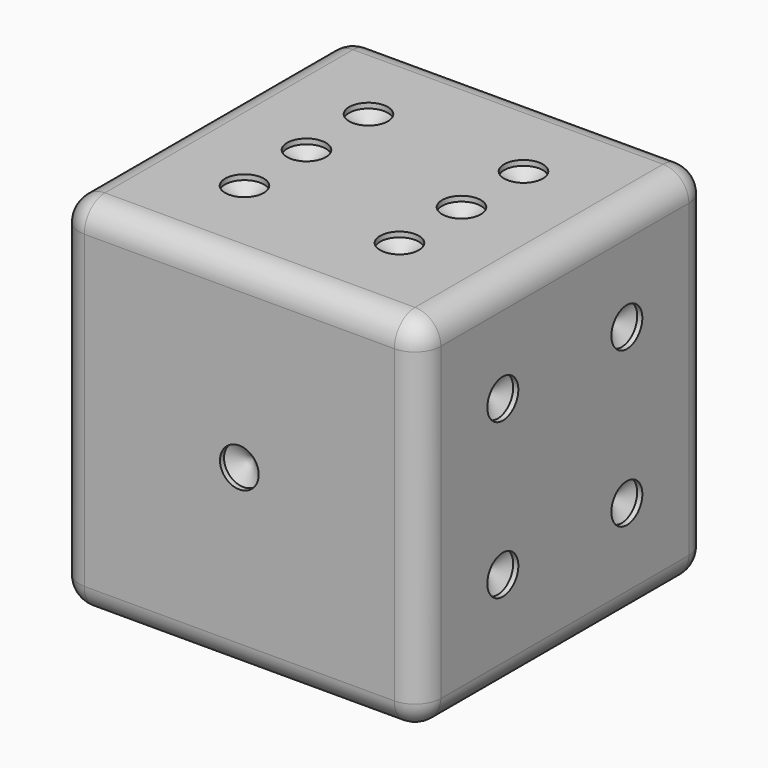
from build123d import *

# Parameters (mm, degrees)
F0_W        = 70
F0_H        = 70
F1_DEPTH    = 35
F2_R        = 5
F3_R        = 5
F4_R        = 5
F5_R        = 5
F6_T1_DEPTH = 77.5
F6_S5_W     = 5
F6_S5_H     = 5
F6_T6_DEPTH = 5
F7_R        = 5
F9_D        = 7.5
F9_DEPTH    = 1
F9_TIP      = 2.2532273214
F11_D       = 7.5
F11_DEPTH   = 1
F11_TIP     = 2.2532273214
F13_D       = 7.5
F13_DEPTH   = 1
F13_TIP     = 2.2532273214
F15_D       = 7.5
F15_DEPTH   = 1
F15_TIP     = 2.2532273214
F17_D       = 7.5
F17_DEPTH   = 1
F17_TIP     = 2.2532273214
F19_D       = 7.5
F19_DEPTH   = 1
F19_TIP     = 2.2532273214


# Not quite as in the source:
# - a fillet or chamfer that OpenCascade refuses, or shapes differently, is made with other operations: its cross-section is extruded or revolved along the edge and cut away or added


with BuildPart() as f1:
    # F0 (on Front) → F1 (new body, symmetric)
    with BuildSketch(Plane.XZ):
        Rectangle(F0_W, F0_H)
    extrude(amount=F1_DEPTH, both=True)

    # F2
    f2_edges = [f1.edges().sort_by_distance(p)[0] for p in [
        (0, 35, -35),
    ]]
    fillet(f2_edges, radius=F2_R)

    # F3
    f3_edges = [f1.edges().sort_by_distance(p)[0] for p in [
        (0, 35, 35),
    ]]
    fillet(f3_edges, radius=F3_R)

    # F4
    f4_edges = [f1.edges().sort_by_distance(p)[0] for p in [
        (0, -35, -35),
    ]]
    fillet(f4_edges, radius=F4_R)

    # F5
    f5_edges = [f1.edges().sort_by_distance(p)[0] for p in [
        (-35, -2.5, 35),
    ]]
    fillet(f5_edges, radius=F5_R)

    # F6: fillet of radius 5 on 1 edges, made by hand

    # F6_s2 → F6_t1 (cut)
    with BuildSketch(Plane.YZ.offset(-30)):
        with BuildLine():
            ThreePointArc((-35, 30), (-33.5355339059, 33.5355339059), (-30, 35))
            Line((-30, 35), (-35, 35))
            Line((-35, 35), (-35, 30))
        make_face()
    extrude(amount=F6_T1_DEPTH, mode=Mode.SUBTRACT)


with BuildPart() as f6_tool4:
    # F6_s5 → F6_t6 (new body)
    with BuildSketch(Plane.XZ.offset(30)):
        with Locations((-32.5, 32.5)):
            Rectangle(F6_S5_W, F6_S5_H)
    extrude(amount=F6_T6_DEPTH)

    # F6_s7 → F6_t8 (revolve, cut)
    with BuildSketch(Plane(origin=(-30, -30, 30), x_dir=(0.7071067812, 0, -0.7071067812), z_dir=(-0.7071067812, 0, -0.7071067812))):
        with BuildLine():
            ThreePointArc((0, -5), (5, 0), (0, 5))
            Line((0, 5), (0, -5))
        make_face()
    revolve(axis=Axis((-30, -30, 30), (0, -1, 0)), mode=Mode.SUBTRACT)


with BuildPart() as f1_1:
    add(f1.part)

    # F6_t3: cut F6_tool4
    add(f6_tool4.part, mode=Mode.SUBTRACT)

    # F7
    f7_edges = [f1_1.edges().sort_by_distance(p)[0] for p in [
        (35, 0, 35),
    ]]
    fillet(f7_edges, radius=F7_R)

    # F9
    with Locations(Plane.XZ.offset(35)):
        with Locations((0, 0)):
            Hole(F9_D / 2, depth=F9_DEPTH)
            with Locations((0, 0, -(F9_DEPTH + F9_TIP / 2))):  # 118° drill point
                Cone(0, F9_D / 2, F9_TIP, mode=Mode.SUBTRACT)

    # F11
    with Locations(Plane.YZ.offset(35)):
        with Locations((-15, 15), (15, 15), (15, -15), (-15, -15)):
            Hole(F11_D / 2, depth=F11_DEPTH)
            with Locations((0, 0, -(F11_DEPTH + F11_TIP / 2))):  # 118° drill point
                Cone(0, F11_D / 2, F11_TIP, mode=Mode.SUBTRACT)

    # F13
    with Locations(Plane.XY.offset(35)):
        with Locations((-15, 15), (15, 15), (15, 0), (15, -15), (-15, -15), (-15, 0)):
            Hole(F13_D / 2, depth=F13_DEPTH)
            with Locations((0, 0, -(F13_DEPTH + F13_TIP / 2))):  # 118° drill point
                Cone(0, F13_D / 2, F13_TIP, mode=Mode.SUBTRACT)

    # F15
    with Locations(Plane(origin=(-35, 0, 0), x_dir=(0, -1, 0), z_dir=(-1, 0, 0))):
        with Locations((-15, -15), (-15, 15), (0, 0), (15, 15), (15, -15)):
            Hole(F15_D / 2, depth=F15_DEPTH)
            with Locations((0, 0, -(F15_DEPTH + F15_TIP / 2))):  # 118° drill point
                Cone(0, F15_D / 2, F15_TIP, mode=Mode.SUBTRACT)

    # F17
    with Locations(Plane(origin=(0, 0, -35), x_dir=(1, 0, 0), z_dir=(0, 0, -1))):
        with Locations((15, -15), (0, 0), (-15, 15)):
            Hole(F17_D / 2, depth=F17_DEPTH)
            with Locations((0, 0, -(F17_DEPTH + F17_TIP / 2))):  # 118° drill point
                Cone(0, F17_D / 2, F17_TIP, mode=Mode.SUBTRACT)

    # F19
    with Locations(Plane(origin=(0, 35, 0), x_dir=(-1, 0, 0), z_dir=(0, 1, 0))):
        with Locations((-15, 15), (15, -15)):
            Hole(F19_D / 2, depth=F19_DEPTH)
            with Locations((0, 0, -(F19_DEPTH + F19_TIP / 2))):  # 118° drill point
                Cone(0, F19_D / 2, F19_TIP, mode=Mode.SUBTRACT)


solid = f1_1.part
